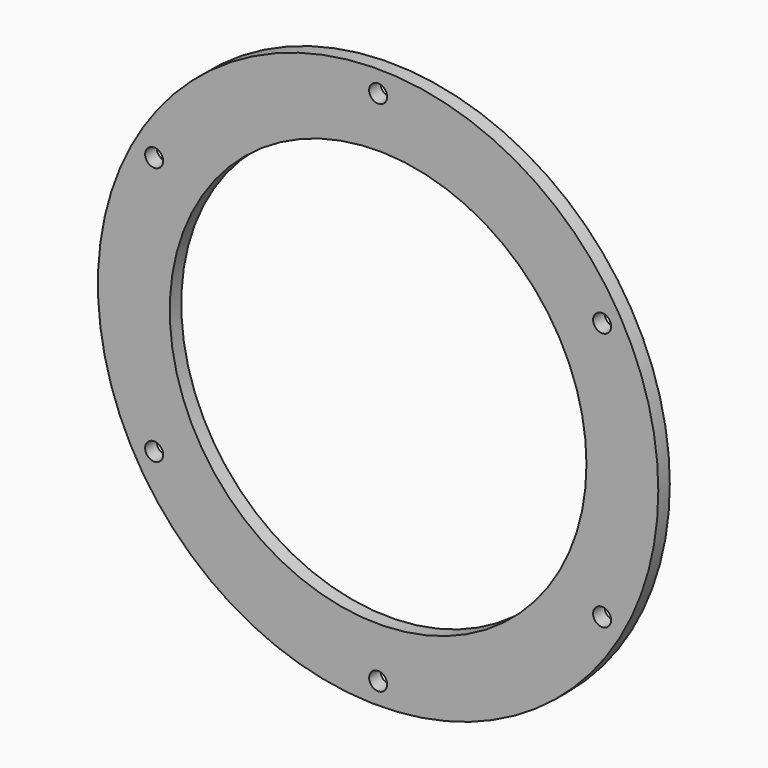
from build123d import *

# Parameters (mm, degrees)
F0_R            = 39
F0_R_2          = 29
F1_DEPTH        = 2
F2_R            = 1.25
F3_DEPTH        = 2.001
F3_COPIES_COUNT = 6


# Not quite as in the source:
# - a pattern or mirror of a feature is missing from the dataset's text; its kind, count and spacing are read off the source's solid


with BuildPart() as f1:
    # F0 (on Front) → F1 (new body)
    with BuildSketch(Plane.XZ):
        Circle(F0_R)
        Circle(F0_R_2, mode=Mode.SUBTRACT)
    extrude(amount=F1_DEPTH)

    # F2 (on face) → F3 (cut, through all)
    with BuildSketch(Plane.XZ.offset(2)):
        with Locations((31.1769145362, 18)):
            Circle(F2_R)
    f3 = extrude(amount=-F3_DEPTH, mode=Mode.SUBTRACT)

    # F3_copies: F3 ×6 about axis
    f3_copies_axis = Axis((0, 0, 0), (0, 1, 0))
    for i in range(1, F3_COPIES_COUNT):
        add(f3.rotate(f3_copies_axis, i * 360 / F3_COPIES_COUNT), mode=Mode.SUBTRACT)


solid = f1.part
